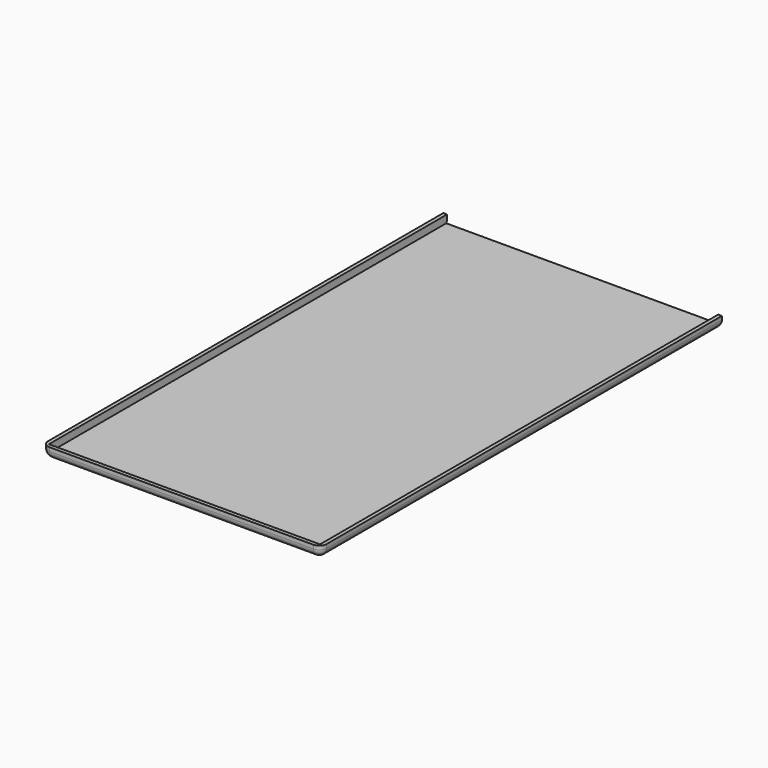
from build123d import *

# Parameters (mm, degrees)
F1_DEPTH     = 3
F0_W         = 73
F0_H         = 134
F2_DEPTH     = 1
F3_T1_DEPTH  = 145
F3_T3_DEPTH  = 85
F4_T1_DEPTH  = 6
F4_S5_W      = 2
F4_S5_H      = 2
F4_T6_DEPTH  = 2
F4_S11_W     = 2
F4_S11_H     = 2
F4_T12_DEPTH = 2


# Not quite as in the source:
# - a fillet or chamfer that OpenCascade refuses, or shapes differently, is made with other operations: its cross-section is extruded or revolved along the edge and cut away or added


with BuildPart() as f1:
    # F0 (on Top) → F1 (new body)
    with BuildSketch(Plane.XY):
        Polygon((0, 135), (0, 0), (75, 0), (75, 135), (74, 135), (74, 1), (1, 1), (1, 135), align=None)
    extrude(amount=F1_DEPTH)

    # F0 (on Top) → F2 (join)
    with BuildSketch(Plane.XY):
        with Locations((37.5, 68)):
            Rectangle(F0_W, F0_H)
    extrude(amount=F2_DEPTH)

    # F3: fillet of radius 2 on 4 edges, made by hand

    # F3_s2 → F3_t1 (cut)
    with BuildSketch(Plane.XZ.offset(-140)):
        with BuildLine():
            ThreePointArc((0, 2), (0.5857864376, 0.5857864376), (2, 0))
            Line((2, 0), (0, 0))
            Line((0, 0), (0, 2))
        make_face()
        with BuildLine():
            ThreePointArc((75, 2), (74.4142135624, 0.5857864376), (73, 0))
            Line((73, 0), (75, 0))
            Line((75, 0), (75, 2))
        make_face()
    extrude(amount=F3_T1_DEPTH, mode=Mode.SUBTRACT)

    # F3_s4 → F3_t3 (cut)
    with BuildSketch(Plane.YZ.offset(-5)):
        with BuildLine():
            ThreePointArc((2, 0), (0.5857864376, 0.5857864376), (0, 2))
            Line((0, 2), (0, 0))
            Line((0, 0), (2, 0))
        make_face()
        with BuildLine():
            ThreePointArc((133, 0), (134.4142135624, 0.5857864376), (135, 2))
            Line((135, 2), (135, 0))
            Line((135, 0), (133, 0))
        make_face()
    extrude(amount=F3_T3_DEPTH, mode=Mode.SUBTRACT)

    # F4: fillet of radius 2 on 2 edges, made by hand

    # F4_s2 → F4_t1 (cut)
    with BuildSketch(Plane.XY.offset(2)):
        with BuildLine():
            ThreePointArc((73, 0), (74.4142135624, 0.5857864376), (75, 2))
            Line((75, 2), (75, 0))
            Line((75, 0), (73, 0))
        make_face()
        with BuildLine():
            ThreePointArc((0, 2), (0.5857864376, 0.5857864376), (2, 0))
            Line((2, 0), (0, 0))
            Line((0, 0), (0, 2))
        make_face()
    extrude(amount=F4_T1_DEPTH, mode=Mode.SUBTRACT)


with BuildPart() as f4_tool4:
    # F4_s5 → F4_t6 (new body)
    with BuildSketch(Plane.YZ.offset(2)):
        with Locations((1, 1)):
            Rectangle(F4_S5_W, F4_S5_H)
    extrude(amount=-F4_T6_DEPTH)

    # F4_s7 → F4_t8 (revolve, cut)
    with BuildSketch(Plane(origin=(2, 2, 2), x_dir=(0, 0.7071067812, 0.7071067812), z_dir=(0, -0.7071067812, 0.7071067812))):
        with BuildLine():
            ThreePointArc((0, -2), (2, 0), (0, 2))
            Line((0, 2), (0, -2))
        make_face()
    revolve(axis=Axis((2, 2, 2), (-1, 0, 0)), mode=Mode.SUBTRACT)


with BuildPart() as f1_1:
    add(f1.part)

    # F4_t3: cut F4_tool4
    add(f4_tool4.part, mode=Mode.SUBTRACT)


with BuildPart() as f4_tool10:
    # F4_s11 → F4_t12 (new body)
    with BuildSketch(Plane.XZ.offset(-2)):
        with Locations((74, 1)):
            Rectangle(F4_S11_W, F4_S11_H)
    extrude(amount=F4_T12_DEPTH)

    # F4_s13 → F4_t14 (revolve, cut)
    with BuildSketch(Plane(origin=(73, 2, 2), x_dir=(-0.7071067812, 0, 0.7071067812), z_dir=(0.7071067812, 0, 0.7071067812))):
        with BuildLine():
            ThreePointArc((0, -2), (2, 0), (0, 2))
            Line((0, 2), (0, -2))
        make_face()
    revolve(axis=Axis((73, 2, 2), (0, -1, 0)), mode=Mode.SUBTRACT)


with BuildPart() as f1_2:
    add(f1_1.part)

    # F4_t9: cut F4_tool10
    add(f4_tool10.part, mode=Mode.SUBTRACT)


solid = f1_2.part
